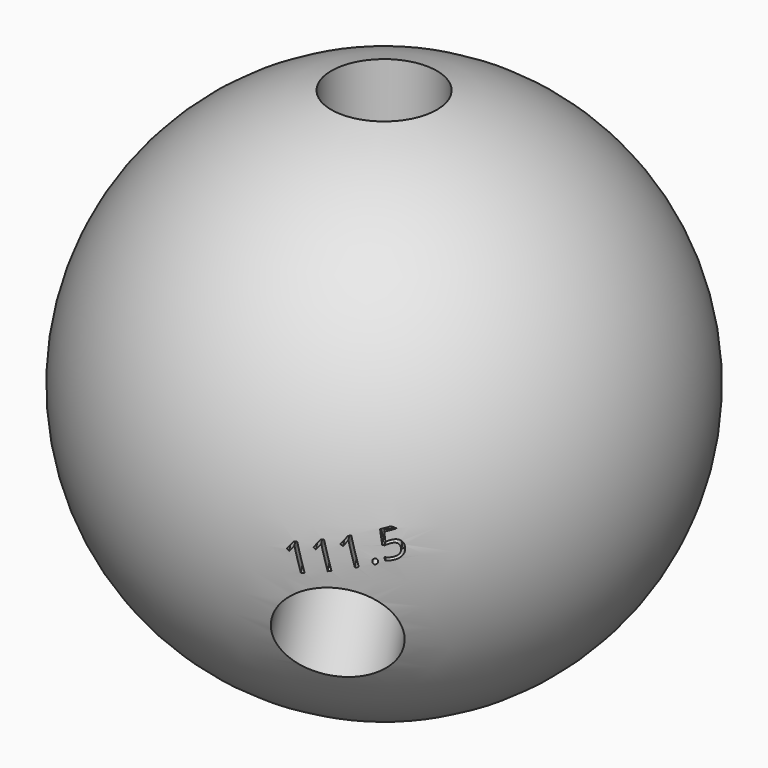
from build123d import *

# Parameters (mm, degrees)
F4_R          = 3.175
F5_DEPTH      = 50.8
F7_ANGLE      = 120
F8_ANGLE      = 111.2
F9_ANGLE      = 120
F10_ANGLE     = -111.5
F11_ANGLE     = -60
F13_TEXT_SIZE = 1.3579025916
F14_DEPTH     = 11.0998
F17_TEXT_SIZE = 2.3087130911
F18_DEPTH     = 4.7752
F19_TEXT_SIZE = 1.8683569376
F20_DEPTH     = 7.0612


# Not quite as in the source:
# - Text() gives the source's letters only with a copy of the font that has no kerning and outlines rounded to 1/6400 em; it was checked with that copy


with BuildPart() as f2:
    # F0 (on Front) → F2 (revolve)
    with BuildSketch(Plane.XZ):
        with BuildLine():
            Line((0, -15.875), (0, 15.875))
            ThreePointArc((0, 15.875), (-15.875, 0), (0, -15.875))
        make_face()
    revolve(axis=Axis((0, 0, 0), (0, 0, 1)))

    # F13 (on offset) → F14 (cut)
    with BuildSketch(Plane(origin=(-23.6810245509, 0, -9.1852640801), x_dir=(0, -1, 0), z_dir=(-0.9323238012, 0, -0.3616245701))):
        with Locations((-2.0063980483, 3.8888063282)):
            Text('111.2', F13_TEXT_SIZE, font='Open Sans', text_align=(TextAlign.LEFT, TextAlign.BOTTOM))
    extrude(amount=-F14_DEPTH, mode=Mode.SUBTRACT)

    # F17 (on offset) → F18 (cut)
    with BuildSketch(Plane(origin=(8.862227335, -15.3498280125, -6.9818483691), x_dir=(0.885200987, 0.4234621037, 0.1926111612), z_dir=(0.465208784, -0.80576525, -0.3665012267))):
        with Locations((-1.368867117, 4.0490613319)):
            Text('111.5', F17_TEXT_SIZE, font='Open Sans', text_align=(TextAlign.LEFT, TextAlign.BOTTOM))
    extrude(amount=-F18_DEPTH, mode=Mode.SUBTRACT)

    # F19 (on offset) → F20 (cut)
    with BuildSketch(Plane(origin=(8.8803842066, 15.3812766365, -6.8889480601), x_dir=(-0.8846994306, 0.4254401089, -0.1905456148), z_dir=(0.4661619006, 0.8074160964, -0.3616245701))):
        with Locations((-2.0978951361, 3.8909006398)):
            Text('111.2', F19_TEXT_SIZE, font='Open Sans', text_align=(TextAlign.LEFT, TextAlign.BOTTOM))
    extrude(amount=-F20_DEPTH, mode=Mode.SUBTRACT)


with BuildPart() as f5:
    # F4 (on offset) → F5 (new body)
    with BuildSketch(Plane.XY.offset(6.35)):
        Circle(F4_R)
    extrude(amount=F5_DEPTH)


with BuildPart() as f7_1:
    # F7: copy of F5
    add(f5.part.rotate(Axis((0, 0, 6.35), (0, 0, -1)), F7_ANGLE))


with BuildPart() as f5_1:
    # F8: moved
    add(f5.part.rotate(Axis((0, -21.7784233391, 0), (0, -1, 0)), F8_ANGLE))


with BuildPart() as f9_1:
    # F9: copy of F5
    add(f5_1.part.rotate(Axis((0, 0, -15.9466937184), (0, 0, -1)), F9_ANGLE))


with BuildPart() as f10_1:
    # F10: copy of F7_1
    add(f7_1.part.rotate(Axis((0, -21.7784233391, 0), (0, -1, 0)), F10_ANGLE))


with BuildPart() as f10_1_1:
    # F11: moved
    add(f10_1.part.rotate(Axis((0, 0, 25.4038926214), (0, 0, 1)), F11_ANGLE))


with BuildPart() as f2_1:
    add(f2.part)

    # F21: cut F7_1, F10_1, F9_1, F5
    add(f7_1.part, mode=Mode.SUBTRACT)
    add(f10_1_1.part, mode=Mode.SUBTRACT)
    add(f9_1.part, mode=Mode.SUBTRACT)
    add(f5_1.part, mode=Mode.SUBTRACT)


solid = f2_1.part
